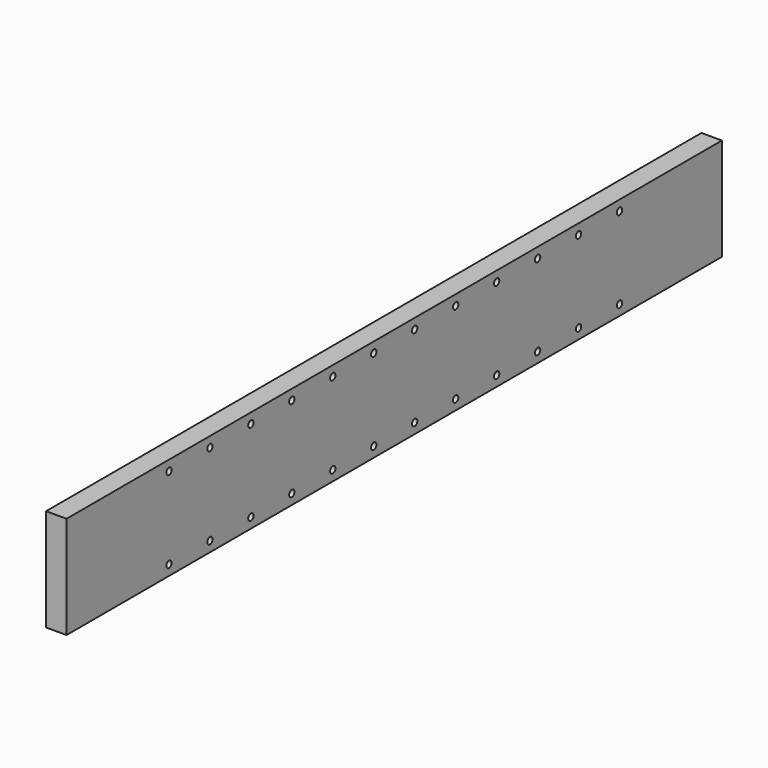
from build123d import *

# Parameters (mm, degrees)
F0_W     = 20
F0_H     = 100
F1_DEPTH = 800
F2_R     = 3.25
F3_DEPTH = 20


# Not quite as in the source:
# - a feature names something its author has since deleted; it is built from what else it names


with BuildPart() as f1:
    # F0 (on Front) → F1 (new body)
    with BuildSketch(Plane.XZ):
        Rectangle(F0_W, F0_H)
    extrude(amount=-F1_DEPTH)

    # F2 (on face) → F3 (cut, through all)
    with BuildSketch(Plane(origin=(-10, 0, 0), x_dir=(0, -1, 0), z_dir=(-1, 0, 0))):
        with Locations((-625, 40)):
            Circle(F2_R)
        with Locations((-575, 40)):
            Circle(F2_R)
        with Locations((-675, 40)):
            Circle(F2_R)
        with Locations((-675, -40)):
            Circle(F2_R)
        with Locations((-625, -40)):
            Circle(F2_R)
        with Locations((-525, -40)):
            Circle(F2_R)
        with Locations((-575, -40)):
            Circle(F2_R)
        with Locations((-525, 40)):
            Circle(F2_R)
        with Locations((-475, 40)):
            Circle(F2_R)
        with Locations((-425, 40)):
            Circle(F2_R)
        with Locations((-375, 40)):
            Circle(F2_R)
        with Locations((-325, 40)):
            Circle(F2_R)
        with Locations((-275, 40)):
            Circle(F2_R)
        with Locations((-225, 40)):
            Circle(F2_R)
        with Locations((-175, 40)):
            Circle(F2_R)
        with Locations((-175, -40)):
            Circle(F2_R)
        with Locations((-225, -40)):
            Circle(F2_R)
        with Locations((-325, -40)):
            Circle(F2_R)
        with Locations((-375, -40)):
            Circle(F2_R)
        with Locations((-425, -40)):
            Circle(F2_R)
        with Locations((-475, -40)):
            Circle(F2_R)
        with Locations((-275, -40)):
            Circle(F2_R)
        with Locations((-125, -40)):
            Circle(F2_R)
        with Locations((-125, 40)):
            Circle(F2_R)
    extrude(amount=-F3_DEPTH, mode=Mode.SUBTRACT)


solid = f1.part
